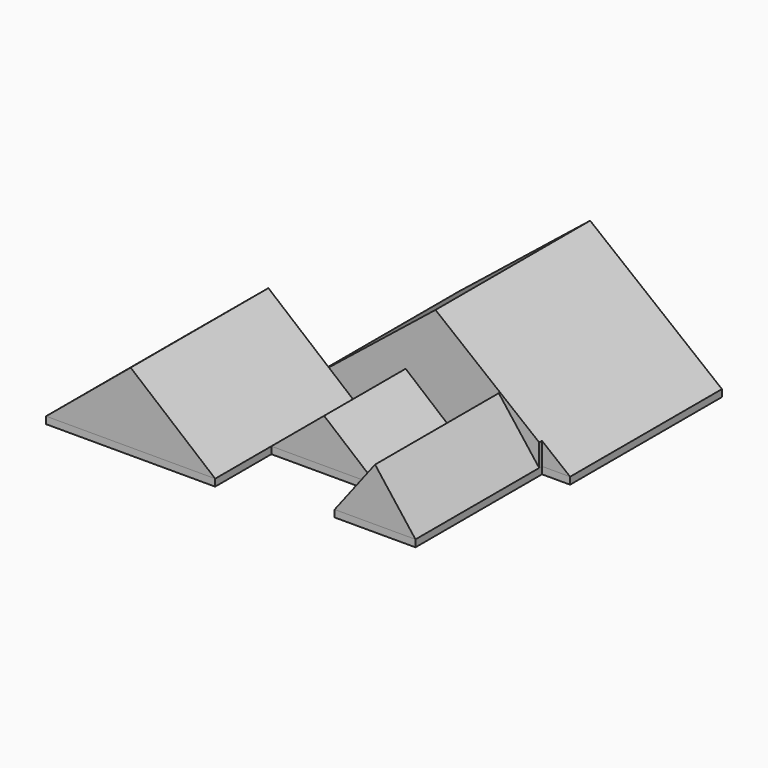
from build123d import *

# Parameters (mm, degrees)
F1_DEPTH  = 50.8
F3_DEPTH  = 50.8
F5_DEPTH  = 508
F7_DEPTH  = 2641.601
F9_DEPTH  = 762
F11_DEPTH = 2641.601
F12_W     = 584.2
F12_H     = 1117.6
F13_DEPTH = 381
F15_DEPTH = 2514.601
F17_DEPTH = 317.5
F19_DEPTH = 2133.601


with BuildPart() as f1:
    # F0 (on Top) → F1 (new body)
    with BuildSketch(Plane.XY):
        Polygon((-962.0625968753, 68.8929493287), (-1444.6625968753, 68.8929493287), (-1774.8625968753, 68.8929493287), (-1774.8625968753, -615.8212534091), (-1774.8625968753, -1175.7070506713), (-1187.7313246546, -1175.7070506713), (-552.7313246546, -1175.7070506713), (-552.7313246546, -667.7070506713), (209.2686753454, -667.7070506713), (209.2686753454, -1048.7070506713), (793.4686753454, -1048.7070506713), (793.4686753454, 94.2929493287), (996.6686753454, 94.2929493287), (996.6686753454, 1465.8929493287), (209.2686753454, 1465.8929493287), (39.6116377057, 1465.8929493287), (-708.0625968753, 1465.8929493287), (-908.3313246546, 1465.8929493287), (-908.3313246546, 957.8929493287), (-908.3313246546, 68.8929493287), align=None)
        Polygon((-606.4625968753, -1123.8212534091), (-1139.8625968753, -1123.8212534091), (-1724.0625968753, -1123.8212534091), (-1724.0625968753, -565.0212534091), (-1721.1313246546, 26.7790361264), (-1441.7313246546, 26.7790361264), (-908.3313246546, 26.7790361264), (-908.3313246546, -515.3070506713), (-784.2625968753, -515.3070506713), (-784.2625968753, -667.7070506713), (-657.2625968753, -667.7070506713), (-606.4625968753, -667.7070506713), align=None, mode=Mode.SUBTRACT)
        Polygon((256.9311268033, -996.8212534091), (256.9311268033, -615.8212534091), (307.7311268033, -615.8212534091), (307.7311268033, -565.0212534091), (256.9311268033, -565.0212534091), (256.9311268033, -361.8212534091), (307.7311268033, -361.8212534091), (307.7311268033, -311.0212534091), (256.9311268033, -311.0212534091), (206.1311268033, -311.0212534091), (206.1311268033, -361.8212534091), (206.1311268033, -615.8212534091), (-98.6688731967, -615.8212534091), (-606.4625968753, -615.8212534091), (-733.4625968753, -615.8212534091), (-733.4625968753, -463.4212534091), (-860.4625968753, -463.4212534091), (-860.4625968753, 19.1787465909), (-702.1286356269, 19.1787465909), (-702.1286356269, 69.9787465909), (-860.4625968753, 69.9787465909), (-860.4625968753, 908.1787465909), (-708.0625968753, 908.1787465909), (-708.0625968753, 957.8929493287), (-860.4625968753, 957.8929493287), (-860.4625968753, 1415.0929493287), (-708.0625968753, 1415.0929493287), (39.6116377057, 1416.1787465909), (192.0116377057, 1416.1787465909), (192.0116377057, 957.8929493287), (39.6116377057, 957.8929493287), (39.6116377057, 908.1787465909), (192.0116377057, 908.1787465909), (192.0116377057, 833.6035154203), (460.3374031247, 833.6035154203), (460.3374031247, 884.4035154203), (256.9311268033, 884.4035154203), (256.9311268033, 1416.1787465909), (942.7311268033, 1416.1787465909), (942.7311268033, 884.4035154203), (574.6374031247, 884.4035154203), (574.6374031247, 833.6035154203), (574.6374031247, 757.4035154203), (625.4374031247, 757.4035154203), (625.4374031247, 833.6035154203), (942.7311268033, 833.6035154203), (942.7311268033, 605.0035154203), (625.4374031247, 605.0035154203), (625.4374031247, 681.2035154203), (574.6374031247, 681.2035154203), (574.6374031247, 605.0035154203), (574.6374031247, 554.2035154203), (942.7311268033, 554.2035154203), (942.7311268033, 146.1787465909), (688.7311268033, 146.1787465909), (256.9311268033, 146.1787465909), (256.9311268033, 554.2035154203), (460.3374031247, 554.2035154203), (460.3374031247, 605.0035154203), (206.1311268033, 605.0035154203), (206.1311268033, 450.9787465909), (206.1311268033, 196.9787465909), (206.1311268033, 146.1787465909), (206.1311268033, 69.9787465909), (53.7311268033, 69.9787465909), (-99.8755003749, 69.9787465909), (-252.2755003749, 69.9787465909), (-252.2755003749, 19.1787465909), (-150.6755003749, 19.1787465909), (-150.6755003749, -82.4212534091), (-99.8755003749, -82.4212534091), (-99.8755003749, 19.1787465909), (53.7311268033, 19.1787465909), (206.1311268033, 19.1787465909), (206.1311268033, -6.2138557284), (206.1311268033, -184.0212534091), (206.1311268033, -209.4212534091), (-99.8755003749, -209.4212534091), (-150.6755003749, -209.4212534091), (-150.6755003749, -311.0212534091), (-201.4755003749, -311.0212534091), (-252.2755003749, -311.0212534091), (-252.2755003749, -361.8212534091), (-99.8755003749, -361.8212534091), (-99.8755003749, -311.0212534091), (-99.8755003749, -260.2212534091), (206.1311268033, -260.2212534091), (256.9311268033, -260.2212534091), (307.7311268033, -260.2212534091), (307.7311268033, -209.4212534091), (256.9311268033, -209.4212534091), (256.9311268033, -158.6212534091), (256.9311268033, 95.3787465909), (688.7311268033, 95.3787465909), (739.5311268033, 95.3787465909), (739.5311268033, -209.4212534091), (739.5311268033, -312.485956351), (739.5311268033, -374.5110579631), (739.5311268033, -615.8212534091), (739.5311268033, -996.8212534091), align=None, mode=Mode.SUBTRACT)
    extrude(amount=F1_DEPTH)


with BuildPart() as f1b:
    # F0 (on Top) → F1, piece 2 (new body)
    with BuildSketch(Plane.XY):
        Polygon((-557.0755003749, -361.8212534091), (-404.6755003749, -361.8212534091), (-404.6755003749, -311.0212534091), (-506.2755003749, -311.0212534091), (-506.2755003749, 19.1787465909), (-404.6755003749, 19.1787465909), (-404.6755003749, 69.9787465909), (-557.0755003749, 69.9787465909), (-557.0755003749, 19.1787465909), (-557.0755003749, -311.0212534091), align=None)
    extrude(amount=F1_DEPTH)


with BuildPart() as f3:
    # F2 (on face) → F3 (new body)
    with BuildSketch(Plane(origin=(0, 0, 0), x_dir=(1, 0, 0), z_dir=(0, 0, -1))):
        Polygon((-552.7313246546, 1175.7070506713), (-1774.8625968753, 1175.7070506713), (-1774.8625968753, -68.8929493287), (-908.3313246546, -68.8929493287), (-908.3313246546, -1465.8929493287), (996.6686753454, -1465.8929493287), (996.6686753454, -94.2929493287), (793.4686753454, -94.2929493287), (793.4686753454, 1048.7070506713), (209.2686753454, 1048.7070506713), (209.2686753454, 667.7070506713), (-552.7313246546, 667.7070506713), align=None)
    extrude(amount=-F3_DEPTH)


with BuildPart() as f5:
    # F4 (on face) → F5 (new body)
    with BuildSketch(Plane.XY.offset(50.8)):
        Polygon((-1774.8625968753, 68.8929493287), (-1774.8625968753, -1175.7070506713), (-552.7313246546, -1175.7070506713), (-552.7313246546, -667.7070506713), (-552.7313246546, 68.8929493287), (-908.3313246546, 68.8929493287), align=None)
    extrude(amount=F5_DEPTH)

    # F6 (on face) → F7 (cut, through all)
    with BuildSketch(Plane.XZ.offset(1175.7070506713)):
        Polygon((-1774.8625968753, 558.8), (-1774.8625968753, 50.8), (-1163.796960765, 558.8), align=None)
        Polygon((-552.7313246546, 558.8), (-1163.796960765, 558.8), (-552.7313246546, 50.8), align=None)
    extrude(amount=-F7_DEPTH, mode=Mode.SUBTRACT)


with BuildPart() as f9:
    # F8 (on face) → F9 (new body)
    with BuildSketch(Plane.XY.offset(50.8)):
        Polygon((-908.3313246546, 1465.8929493287), (-908.3313246546, 68.8929493287), (793.4686753454, 68.8929493287), (793.4686753454, 94.2929493287), (996.6686753454, 94.2929493287), (996.6686753454, 1465.8929493287), align=None)
    extrude(amount=F9_DEPTH)

    # F10 (on face) → F11 (cut, through all)
    with BuildSketch(Plane(origin=(0, 1465.8929493287, 0), x_dir=(-1, 0, 0), z_dir=(0, 1, 0))):
        Polygon((-996.6686753454, 812.8), (-996.6686753454, 50.8), (-44.1686753454, 812.8), align=None)
        Polygon((908.3313246546, 812.8), (-44.1686753454, 812.8), (908.3313246546, 50.8), align=None)
    extrude(amount=-F11_DEPTH, mode=Mode.SUBTRACT)


with BuildPart() as f13:
    # F12 (on face) → F13 (new body)
    with BuildSketch(Plane.XY.offset(50.8)):
        with Locations((501.3686753454, -489.9070506713)):
            Rectangle(F12_W, F12_H)
    extrude(amount=F13_DEPTH)

    # F14 (on face) → F15 (cut, through all)
    with BuildSketch(Plane.XZ.offset(1048.7070506713)):
        Polygon((209.2686753454, 431.8), (209.2686753454, 50.8), (501.3686753454, 431.8), align=None)
        Polygon((793.4686753454, 431.8), (501.3686753454, 431.8), (793.4686753454, 50.8), align=None)
    extrude(amount=-F15_DEPTH, mode=Mode.SUBTRACT)


with BuildPart() as f17:
    # F16 (on face) → F17 (new body)
    with BuildSketch(Plane.XY.offset(50.8)):
        Polygon((-552.7313246546, 68.8929493287), (-552.7313246546, -667.7070506713), (209.2686753454, -667.7070506713), (209.2686753454, 68.8929493287), (44.1686753454, 68.8929493287), align=None)
    extrude(amount=F17_DEPTH)

    # F18 (on face) → F19 (cut, through all)
    with BuildSketch(Plane.XZ.offset(667.7070506713)):
        Polygon((-552.7313246546, 368.3), (-552.7313246546, 50.8), (-171.7313246546, 368.3), align=None)
        Polygon((209.2686753454, 368.3), (-171.7313246546, 368.3), (209.2686753454, 50.8), align=None)
    extrude(amount=-F19_DEPTH, mode=Mode.SUBTRACT)


solid = Compound([f1.part, f1b.part, f3.part, f5.part, f9.part, f13.part, f17.part])
